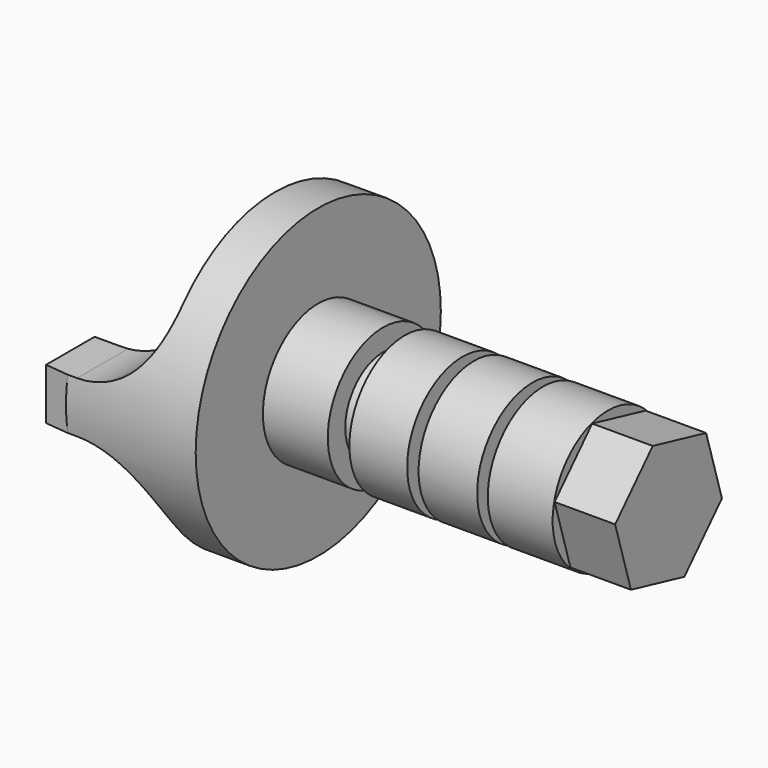
from build123d import *
from build123d import SkipClean  # not in build123d's __all__

# Parameters (mm, degrees)
F0_R      = 45
F1_DEPTH  = 38.1
F2_R      = 13.9074924411
F3_DEPTH  = 92.41422
F7_R      = 20.32
F8_DEPTH  = 19.05
F9_R      = 20.32
F10_DEPTH = 16.96493
F11_R     = 20.32
F12_DEPTH = 17.20109
F13_R     = 20.32
F14_DEPTH = 19.05
F16_DEPTH = 17.78
F17_W     = 88.86107839
F17_H     = 39.3804269531
F18_DEPTH = 25.4
F19_R     = 22.6323588882
F23_DEPTH = 6.92853
F24_W     = 6.92853
F24_H     = 2.8661746596
F25_DEPTH = 25.4


with BuildPart() as f1:
    # F0 (on Right) → F1 (new body)
    with BuildSketch(Plane.YZ):
        Circle(F0_R)
    extrude(amount=-F1_DEPTH)

    # F2 (on face) → F3 (join)
    with BuildSketch(Plane.YZ):
        Circle(F2_R)
    extrude(amount=F3_DEPTH)

    # F7 (on Right) → F8 (join)
    with BuildSketch(Plane.YZ):
        Circle(F7_R)
    extrude(amount=F8_DEPTH)

    # F9 (on offset) → F10 (join)
    with BuildSketch(Plane.YZ.offset(25.4)):
        Circle(F9_R)
    extrude(amount=F10_DEPTH)

    # F11 (on offset) → F12 (join)
    with BuildSketch(Plane.YZ.offset(45.72)):
        Circle(F11_R)
    extrude(amount=F12_DEPTH)

    # F13 (on offset) → F14 (join)
    with BuildSketch(Plane.YZ.offset(66.04)):
        Circle(F13_R)
    extrude(amount=F14_DEPTH)

    # F15 (on face) → F16 (join)
    with BuildSketch(Plane.YZ.offset(85.09)):
        Polygon((13.7920507069, 14.6662479487), (-5.8053179483, 19.2773902568), (-19.5973686552, 4.6111423081), (-13.7920507069, -14.6662479487), (5.8053179483, -19.2773902568), (19.5973686552, -4.6111423081), align=None)
    extrude(amount=F16_DEPTH)

    # F17 (on face) → F18 (cut)
    with BuildSketch(Plane(origin=(-38.1, 0, 0), x_dir=(0, -1, 0), z_dir=(-1, 0, 0))):
        with Locations((0.0670028883, 27.2318741928)):
            Rectangle(F17_W, F17_H)
        with Locations((0.0670028883, -27.2318741928)):
            Rectangle(F17_W, F17_H)
    extrude(amount=-F18_DEPTH, mode=Mode.SUBTRACT)

    # F19
    f19_edges = [f1.edges().sort_by_distance(p)[0] for p in [
        (-12.7, 0, 7.541661),
        (-12.7, 0, -7.541661),
    ]]
    fillet(f19_edges, radius=F19_R)

    # F20 (on face) → F21 (revolve, cut)
    with BuildSketch(Plane(origin=(-38.1, 0, 0), x_dir=(0, -1, 0), z_dir=(-1, 0, 0))):
        with BuildLine():
            Line((0, -7.5416607163), (0, 0))
            Line((0, 0), (0, 7.5416607163))
            Line((0, 7.5416607163), (-25.8131183102, 7.5416607163))
            ThreePointArc((-25.8131183102, 7.5416607163), (-26.8922614009, 0), (-25.8131183102, -7.5416607163))
            Line((-25.8131183102, -7.5416607163), (0, -7.5416607163))
        make_face()
        with BuildLine():
            Line((-25.8131183102, 7.5416607163), (0, 7.5416607163))
            Line((0, 7.5416607163), (0, 26.8922614009))
            ThreePointArc((0, 26.8922614009), (-16.1304279527, 21.5175049045), (-25.8131183102, 7.5416607163))
        make_face()
        with BuildLine():
            Line((0, -26.8922614009), (0, -7.5416607163))
            Line((0, -7.5416607163), (-25.8131183102, -7.5416607163))
            ThreePointArc((-25.8131183102, -7.5416607163), (-16.1304279527, -21.5175049045), (0, -26.8922614009))
        make_face()
    revolve(axis=Axis((-38.1, 0, 10.4196144343), (0, 0, -1)), mode=Mode.SUBTRACT)

    # F22 (on face) → F23 (join)
    with BuildSketch(Plane(origin=(-38.1, 0, 0), x_dir=(0, -1, 0), z_dir=(-1, 0, 0))):
        with BuildLine():
            Line((-25.8131183102, 7.5416607163), (-44.3635363068, 7.5416607163))
            ThreePointArc((-44.3635363068, 7.5416607163), (-45, 0), (-44.3635363068, -7.5416607163))
            Line((-44.3635363068, -7.5416607163), (-25.8131183102, -7.5416607163))
            ThreePointArc((-25.8131183102, -7.5416607163), (-26.8922614009, 0), (-25.8131183102, 7.5416607163))
        make_face()
        with BuildLine():
            ThreePointArc((25.8131183102, 7.5416607163), (26.8922614009, 0), (25.8131183102, -7.5416607163))
            Line((25.8131183102, -7.5416607163), (44.3635363068, -7.5416607163))
            ThreePointArc((44.3635363068, -7.5416607163), (45, 0), (44.3635363068, 7.5416607163))
            Line((44.3635363068, 7.5416607163), (25.8131183102, 7.5416607163))
        make_face()
    with SkipClean():  # cleaning this boolean's faces spoils the solid; the shape is the same uncleaned
        extrude(amount=F23_DEPTH)

    # F24 (on face) → F25 (cut)
    with BuildSketch(Plane(origin=(0, 0, -7.5416607163), x_dir=(1, 0, 0), z_dir=(0, 0, -1))):
        Polygon((-45.02853, 43.6333455145), (-38.1, 44.3635363068), (-38.1, 47.2297109663), (-45.02853, 47.2297109663), (-45.02853, 44.3635363068), align=None)
        Polygon((-45.02853, -44.3635363068), (-38.1, -44.3635363068), (-45.02853, -43.6333455145), align=None)
        with Locations((-41.564265, -45.7966236366)):
            Rectangle(F24_W, F24_H)
    extrude(amount=-F25_DEPTH, mode=Mode.SUBTRACT)


solid = f1.part
